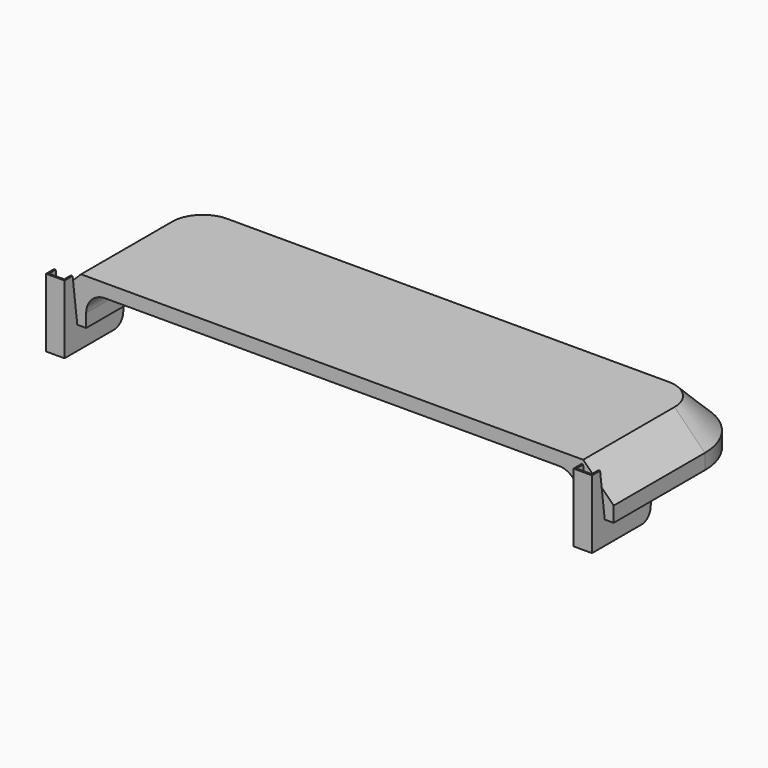
from build123d import *

# Parameters (mm, degrees)
F2_DEPTH      = 12
F3_SIZE       = 8
F0_W          = 14.1
F0_H          = 8.3
F0_W_2        = 40
F4_DEPTH      = 5
F6_DEPTH      = 3
F7_DEPTH      = 20
F7_DEPTH_BACK = 20
F8_START      = 39
F8_DEPTH      = 14.1
F9_START      = -39
F9_DEPTH      = 14.1
F0_W_3        = 4.85
F0_H_2        = 13.3
F10_DEPTH     = 6
F12_DEPTH     = 8.5
F13_W         = 4.85
F13_H         = 5.2
F14_DEPTH     = 6
F15_R         = 2.99999
F16_R         = 5
F17_W         = 5
F17_H         = 8.9
F18_DEPTH     = 5
F20_DEPTH     = 0.8
F21_DEPTH     = 12
F23_DEPTH     = 145.751


# Not quite as in the source:
# - a fillet or chamfer is up to 0.001 mm smaller than in the source, because OpenCascade refuses the exact size


with BuildPart() as f2:
    # F1 (on Top) → F2 (new body)
    with BuildSketch(Plane.XY):
        with BuildLine():
            Line((58, 4), (-58, 4))
            ThreePointArc((-58, 4), (-69.313708499, -0.686291501), (-74, -12))
            Line((-74, -12), (-74, -42))
            Line((-74, -42), (74, -42))
            Line((74, -42), (74, -12))
            ThreePointArc((74, -12), (69.313708499, -0.686291501), (58, 4))
        make_face()
    extrude(amount=F2_DEPTH)

    # F3
    f3_edges = [f2.edges().sort_by_distance(p)[0] for p in [
        (74, -27, 12),
        (0, 4, 12),
        (-74, -27, 12),
    ]]
    chamfer(f3_edges, length=F3_SIZE)

    # F0 (on Top) → F4 (join)
    with BuildSketch(Plane.XY):
        with Locations((-46.05, -4.15)):
            Rectangle(F0_W, F0_H)
        with Locations((0, -4.15)):
            Rectangle(F0_W_2, F0_H)
        with Locations((46.05, -4.15)):
            Rectangle(F0_W, F0_H)
    extrude(amount=-F4_DEPTH)

    # F6 (cut): faces of the model
    f6_faces = [f2.faces().sort_by_distance(p)[0] for p in [
        (0, -8.3, -2.5),
        (46.05, -8.3, -2.5),
        (-46.05, -8.3, -2.5),
    ]]
    extrude(f6_faces, amount=-F6_DEPTH, mode=Mode.SUBTRACT)

    # F5 (on Right) → F7 (join, two sides)
    with BuildSketch(Plane.YZ) as f7_sk:
        Polygon((-5.8, 0), (-8.3, 0), (-8.3, -0.35), (-8.9, -0.55), (-8, -5), (-5.8, -5), align=None)
    extrude(amount=F7_DEPTH)
    extrude(f7_sk.sketch, amount=-F7_DEPTH_BACK)

    # F5 (on Right) → F8 (join)
    with BuildSketch(Plane.YZ.offset(F8_START)):
        Polygon((-5.8, 0), (-8.3, 0), (-8.3, -0.35), (-8.9, -0.55), (-8, -5), (-5.8, -5), align=None)
    extrude(amount=F8_DEPTH)

    # F5 (on Right) → F9 (join)
    with BuildSketch(Plane.YZ.offset(F9_START)):
        Polygon((-5.8, 0), (-8.3, 0), (-8.3, -0.35), (-8.9, -0.55), (-8, -5), (-5.8, -5), align=None)
    extrude(amount=-F9_DEPTH)

    # F0 (on Top) → F10 (join)
    with BuildSketch(Plane.XY):
        with Locations((69.325, -33.65)):
            Rectangle(F0_W_3, F0_H_2)
        with Locations((-69.325, -33.65)):
            Rectangle(F0_W_3, F0_H_2)
    extrude(amount=-F10_DEPTH)

    # F11 (on face) → F12 (cut)
    with BuildSketch(Plane(origin=(0, 0, 0), x_dir=(1, 0, 0), z_dir=(0, 0, -1))):
        with BuildLine():
            Line((64.65, 18.9), (64.65, 42))
            Line((64.65, 42), (-64.65, 42))
            Line((-64.65, 42), (-64.65, 18.9))
            ThreePointArc((-64.65, 18.9), (-61.7210678119, 11.8289321881), (-54.65, 8.9))
            Line((-54.65, 8.9), (54.65, 8.9))
            ThreePointArc((54.65, 8.9), (61.7210678119, 11.8289321881), (64.65, 18.9))
        make_face()
    extrude(amount=-F12_DEPTH, mode=Mode.SUBTRACT)

    # F13 (on face) → F14 (join)
    with BuildSketch(Plane.XZ.offset(40.3)):
        with Locations((69.325, -3.4)):
            Rectangle(F13_W, F13_H)
        with Locations((-69.325, -3.4)):
            Rectangle(F13_W, F13_H)
    extrude(amount=F14_DEPTH)

    # F15 (radius 3 in the source; OpenCascade refuses exactly that, so slightly less here)
    f15_edges = [f2.edges().sort_by_distance(p)[0] for p in [
        (0, 0, -5),
        (-46.05, 0, -5),
        (46.05, 0, -5),
        (-69.325, -27, -6),
        (69.325, -27, -6),
        (69.325, -27, 0),
        (-69.325, -27, 0),
    ]]
    fillet(f15_edges, radius=F15_R)

    # F16
    f16_edges = [f2.edges().sort_by_distance(p)[0] for p in [
        (64.65, -30.45, 8.5),
    ]]
    fillet(f16_edges, radius=F16_R)

    # F17 (on face) → F18 (cut, through all)
    with BuildSketch(Plane(origin=(0, 0, -5), x_dir=(1, 0, 0), z_dir=(0, 0, -1))):
        with Locations((0, 4.45)):
            Rectangle(F17_W, F17_H)
    extrude(amount=-F18_DEPTH, mode=Mode.SUBTRACT)

    # F19 (on face) → F20 (join, through all)
    with BuildSketch(Plane.XY.offset(-0.8)):
        Polygon((71.75, -46.3), (71.75, -40.3), (71.35, -40.3), (71.35, -45.9), (67.3, -45.9), (67.3, -40.3), (66.9, -40.3), (66.9, -46.3), align=None)
        Polygon((-71.35, -40.3), (-71.75, -40.3), (-71.75, -46.3), (-66.9, -46.3), (-66.9, -40.3), (-67.3, -40.3), (-67.3, -45.9), (-71.35, -45.9), align=None)
    extrude(amount=F20_DEPTH)

    # F21 (add, through all): faces of the model
    f21_faces = [f2.faces().sort_by_distance(p)[0] for p in [
        (69.325, -46.2351829498, 0),
        (-71.55, -42.0648170502, 0),
    ]]
    extrude(f21_faces, amount=F21_DEPTH)

    # F22 (on face) → F23 (cut, through all)
    with BuildSketch(Plane.YZ.offset(71.75)):
        Polygon((-42, -0.8), (-42, 12.0000000009), (-43.6490774155, 12), align=None)
    extrude(amount=-F23_DEPTH, mode=Mode.SUBTRACT)


solid = f2.part
